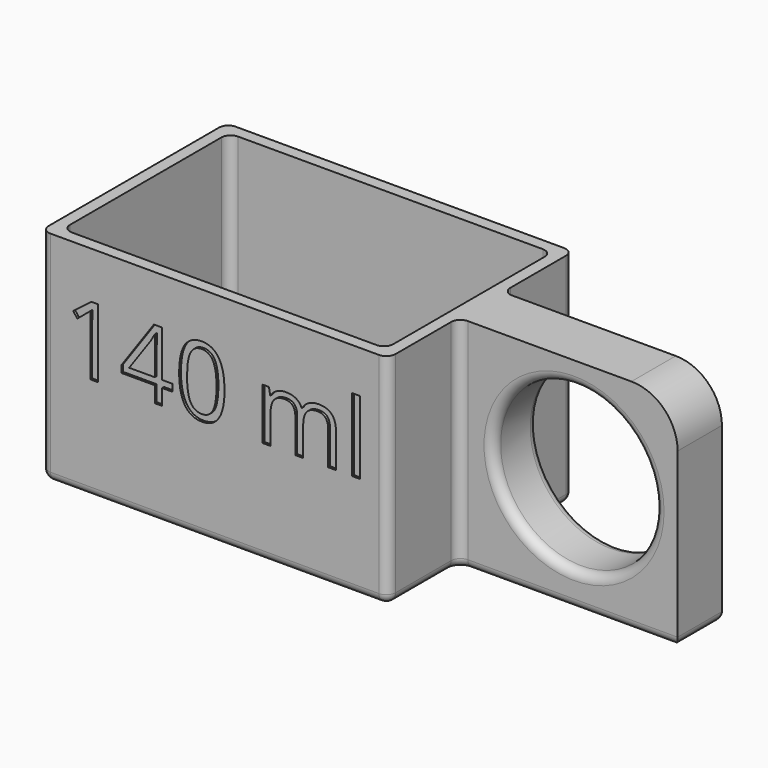
from build123d import *

# Parameters (mm, degrees)
F0_W          = 75.14
F0_H          = 50.14
F0_W_2        = 70
F0_H_2        = 45
F1_DEPTH      = 45
F2_DEPTH      = 2.5
F3_R          = 2
F4_R          = 17.5
F5_DEPTH      = 6
F6_T1_DEPTH   = 47.5
F6_T3_DEPTH   = 15.07
F6_T5_DEPTH   = 50.43
F6_T7_DEPTH   = 22
F6_T9_DEPTH   = 15.07
F6_S13_W      = 2.04
F6_S13_H      = 2.04
F6_T14_DEPTH  = 2.04
F6_S19_W      = 2.04
F6_S19_H      = 2.04
F6_T20_DEPTH  = 2.04
F6_T28_ANGLE  = 90
F6_T30_ANGLE  = 90
F7_TEXT_SIZE  = 20.8333333333
F8_DEPTH      = 0.5
F9_DEPTH      = 0.5
F10_TEXT_SIZE = 20.8333333333
F11_DEPTH     = 0.5


# Not quite as in the source:
# - a fillet or chamfer that OpenCascade refuses, or shapes differently, is made with other operations: its cross-section is extruded or revolved along the edge and cut away or added
# - Text() gives the source's letters only with a copy of the font that has no kerning and outlines rounded to 1/6400 em; it was checked with that copy


with BuildPart() as f1:
    # F0 (on Top) → F1 (new body)
    with BuildSketch(Plane.XY):
        Rectangle(F0_W, F0_H)
        Rectangle(F0_W_2, F0_H_2, mode=Mode.SUBTRACT)
    extrude(amount=F1_DEPTH)

    # F0 (on Top) → F2 (join)
    with BuildSketch(Plane.XY):
        Rectangle(F0_W, F0_H)
        Rectangle(F0_W_2, F0_H_2, mode=Mode.SUBTRACT)
        Rectangle(F0_W_2, F0_H_2)
    extrude(amount=-F2_DEPTH)

    # F3
    f3_edges = [f1.edges().sort_by_distance(p)[0] for p in [
        (-35, 22.5, 22.5),
        (-35, 0, 0),
        (0, 22.5, 0),
        (-35, -22.5, 22.5),
        (35, 22.5, 22.5),
        (35, 0, 0),
        (0, -22.5, 0),
        (35, -22.5, 22.5),
        (37.57, -25.07, 21.25),
        (37.57, 25.07, 21.25),
        (-37.57, -25.07, 21.25),
        (-37.57, 25.07, 21.25),
        (0, -25.07, -2.5),
        (-37.57, 0, -2.5),
        (0, 25.07, -2.5),
    ]]
    fillet(f3_edges, radius=F3_R)

    # F4 (on Front) → F5 (join, symmetric)
    with BuildSketch(Plane.XZ):
        with BuildLine():
            Line((75, 45), (37.57, 45))
            Line((37.57, 45), (37.57, -2.5))
            Line((37.57, -2.5), (85, -2.5))
            Line((85, -2.5), (85, 35))
            ThreePointArc((85, 35), (82.0710678119, 42.0710678119), (75, 45))
        make_face()
        with Locations((62.57, 22.5)):
            Circle(F4_R, mode=Mode.SUBTRACT)
    extrude(amount=F5_DEPTH, both=True)

    # F6: fillet of radius 2 on 9 edges, made by hand

    # F6_s2 → F6_t1 (join)
    with BuildSketch(Plane.XY.offset(-2.5)):
        with BuildLine():
            ThreePointArc((37.57, -8), (38.1557864376, -6.5857864376), (39.57, -6))
            Line((39.57, -6), (37.57, -6))
            Line((37.57, -6), (37.57, -8))
        make_face()
        with BuildLine():
            ThreePointArc((37.57, 8), (38.1557864376, 6.5857864376), (39.57, 6))
            Line((39.57, 6), (37.57, 6))
            Line((37.57, 6), (37.57, 8))
        make_face()
    extrude(amount=F6_T1_DEPTH)

    # F6_s4 → F6_t3 (cut)
    with BuildSketch(Plane.XZ.offset(-23.07)):
        with BuildLine():
            ThreePointArc((37.57, -0.5), (36.9842135624, -1.9142135624), (35.57, -2.5))
            Line((35.57, -2.5), (37.57, -2.5))
            Line((37.57, -2.5), (37.57, -0.5))
        make_face()
    extrude(amount=F6_T3_DEPTH, mode=Mode.SUBTRACT)

    # F6_s6 → F6_t5 (cut)
    with BuildSketch(Plane.YZ.offset(39.57)):
        with BuildLine():
            ThreePointArc((6, -0.5), (5.4142135624, -1.9142135624), (4, -2.5))
            Line((4, -2.5), (6, -2.5))
            Line((6, -2.5), (6, -0.5))
        make_face()
        with BuildLine():
            ThreePointArc((-6, -0.5), (-5.4142135624, -1.9142135624), (-4, -2.5))
            Line((-4, -2.5), (-6, -2.5))
            Line((-6, -2.5), (-6, -0.5))
        make_face()
    extrude(amount=F6_T5_DEPTH, mode=Mode.SUBTRACT)

    # F6_s8 → F6_t7 (cut)
    with BuildSketch(Plane.XZ.offset(-11)):
        with BuildLine():
            ThreePointArc((83, -2.5), (84.4142135624, -1.9142135624), (85, -0.5))
            Line((85, -0.5), (85, -2.5))
            Line((85, -2.5), (83, -2.5))
        make_face()
    extrude(amount=F6_T7_DEPTH, mode=Mode.SUBTRACT)

    # F6_s10 → F6_t9 (cut)
    with BuildSketch(Plane.XZ.offset(8)):
        with BuildLine():
            ThreePointArc((37.57, -0.5), (36.9842135624, -1.9142135624), (35.57, -2.5))
            Line((35.57, -2.5), (37.57, -2.5))
            Line((37.57, -2.5), (37.57, -0.5))
        make_face()
    extrude(amount=F6_T9_DEPTH, mode=Mode.SUBTRACT)


with BuildPart() as f6_tool12:
    # F6_s13 → F6_t14 (new body)
    with BuildSketch(Plane.YZ.offset(35.57)):
        with Locations((-24.09, -1.52)):
            Rectangle(F6_S13_W, F6_S13_H)
    extrude(amount=F6_T14_DEPTH)

    # F6_s15 → F6_t16 (revolve, cut)
    with BuildSketch(Plane(origin=(35.57, -23.07, -0.5), x_dir=(0, 0.7071067812, 0.7071067812), z_dir=(0, 0.7071067812, -0.7071067812))):
        with BuildLine():
            ThreePointArc((0, -2), (2, 0), (0, 2))
            Line((0, 2), (0, -2))
        make_face()
    revolve(axis=Axis((35.57, -23.07, -0.5), (1, 0, 0)), mode=Mode.SUBTRACT)


with BuildPart() as f1_1:
    add(f1.part)

    # F6_t11: cut F6_tool12
    add(f6_tool12.part, mode=Mode.SUBTRACT)


with BuildPart() as f6_tool18:
    # F6_s19 → F6_t20 (new body)
    with BuildSketch(Plane.YZ.offset(35.57)):
        with Locations((24.09, -1.52)):
            Rectangle(F6_S19_W, F6_S19_H)
    extrude(amount=F6_T20_DEPTH)

    # F6_s21 → F6_t22 (revolve, cut)
    with BuildSketch(Plane(origin=(35.57, 23.07, -0.5), x_dir=(0, -0.7071067812, 0.7071067812), z_dir=(0, 0.7071067812, 0.7071067812))):
        with BuildLine():
            ThreePointArc((0, -2), (2, 0), (0, 2))
            Line((0, 2), (0, -2))
        make_face()
    revolve(axis=Axis((35.57, 23.07, -0.5), (1, 0, 0)), mode=Mode.SUBTRACT)


with BuildPart() as f1_2:
    add(f1_1.part)

    # F6_t17: cut F6_tool18
    add(f6_tool18.part, mode=Mode.SUBTRACT)

    # F6_s23 → F6_t24 (revolve, cut)
    with BuildSketch(Plane.XY.offset(22.5)):
        with BuildLine():
            ThreePointArc((82.07, -6), (80.6557864376, -5.4142135624), (80.07, -4))
            Line((80.07, -4), (80.07, -6))
            Line((80.07, -6), (82.07, -6))
        make_face()
    revolve(axis=Axis((62.57, -6, 22.5), (0, -1, 0)), mode=Mode.SUBTRACT)

    # F6_s25 → F6_t26 (revolve, cut)
    with BuildSketch(Plane.XY.offset(22.5)):
        with BuildLine():
            ThreePointArc((82.07, 6), (80.6557864376, 5.4142135624), (80.07, 4))
            Line((80.07, 4), (80.07, 6))
            Line((80.07, 6), (82.07, 6))
        make_face()
    revolve(axis=Axis((62.57, 6, 22.5), (0, -1, 0)), mode=Mode.SUBTRACT)

    # F6_s27 → F6_t28 (revolve, cut)
    with BuildSketch(Plane.XZ.offset(8)):
        with BuildLine():
            ThreePointArc((35.57, -2.5), (36.9842135624, -1.9142135624), (37.57, -0.5))
            Line((37.57, -0.5), (37.57, -2.5))
            Line((37.57, -2.5), (35.57, -2.5))
        make_face()
    revolve(axis=Axis((39.57, -8, -2.5), (0, 0, -1)), revolution_arc=F6_T28_ANGLE, mode=Mode.SUBTRACT)

    # F6_s29 → F6_t30 (revolve, cut)
    with BuildSketch(Plane.XZ.offset(-8)):
        with BuildLine():
            ThreePointArc((35.57, -2.5), (36.9842135624, -1.9142135624), (37.57, -0.5))
            Line((37.57, -0.5), (37.57, -2.5))
            Line((37.57, -2.5), (35.57, -2.5))
        make_face()
    revolve(axis=Axis((39.57, 8, -2.5), (0, 0, 1)), revolution_arc=F6_T30_ANGLE, mode=Mode.SUBTRACT)

    # F7 (on face) → F8 (cut)
    with BuildSketch(Plane.XZ.offset(25.07)):
        with Locations((-32.57, 20)):
            Text('140 ml', F7_TEXT_SIZE, font='Open Sans', text_align=(TextAlign.LEFT, TextAlign.BOTTOM))
    extrude(amount=-F8_DEPTH, mode=Mode.SUBTRACT)

    # F7 (on face) → F9 (cut)
    with BuildSketch(Plane.XZ.offset(25.07)):
        with Locations((-32.57, 20)):
            Text('140 ml', F7_TEXT_SIZE, font='Open Sans', text_align=(TextAlign.LEFT, TextAlign.BOTTOM))
    extrude(amount=-F9_DEPTH, mode=Mode.SUBTRACT)

    # F10 (on face) → F11 (cut)
    with BuildSketch(Plane(origin=(0, 25.07, 0), x_dir=(-1, 0, 0), z_dir=(0, 1, 0))):
        with Locations((-32.57, 20)):
            Text('140 ml', F10_TEXT_SIZE, font='Open Sans', text_align=(TextAlign.LEFT, TextAlign.BOTTOM))
    extrude(amount=-F11_DEPTH, mode=Mode.SUBTRACT)


solid = f1_2.part
